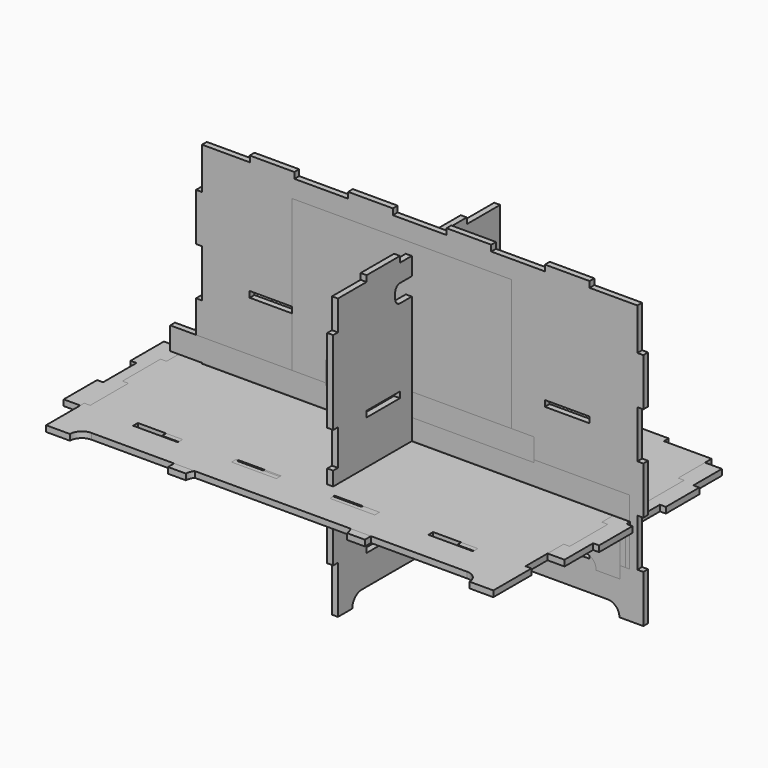
from build123d import *

# Parameters (mm, degrees)
F1_DEPTH  = 12.7
F3_DEPTH  = 12.7
F4_W      = 95.25
F4_H      = 12.7
F4_H_2    = 12.3182607685
F5_DEPTH  = 12.7
F6_W      = 88.9
F6_H      = 12.7
F7_DEPTH  = 12.7
F9_DEPTH  = 12.7
F11_DEPTH = 12.7
F13_DEPTH = 12.7
F14_W     = 88.9
F14_H     = 12.7
F15_DEPTH = 12.7
F16_W     = 95.25
F16_H     = 12.7
F16_H_2   = 12.3182607685
F17_DEPTH = 12.7
F18_W     = 467.36
F18_H     = 482.6
F19_DEPTH = 12.7
F18_W_2   = 15.24
F20_DEPTH = 6.35
F21_W     = 977.9
F21_H     = 48.26
F22_DEPTH = 12.7
F23_W     = 444.5
F23_H     = 48.26
F24_DEPTH = 12.7


with BuildPart() as f1:
    # F0 (on Top) → F1 (new body)
    with BuildSketch(Plane.XY):
        Polygon((-533.4, -256.6132211758), (-520.7, -256.6132211758), (-419.1, -256.6132211758), (-419.1, -243.9132211758), (-323.85, -243.9132211758), (-323.85, -256.6132211758), (-209.55, -256.6132211758), (-209.55, -243.9132211758), (-114.3, -243.9132211758), (-114.3, -256.6132211758), (0, -256.6132211758), (0, -243.9132211758), (95.25, -243.9132211758), (95.25, -256.6132211758), (209.55, -256.6132211758), (209.55, -243.9132211758), (304.8, -243.9132211758), (304.8, -256.6132211758), (406.4, -256.6132211758), (419.1, -256.6132211758), (419.1, -167.7132211758), (406.4, -167.7132211758), (406.4, -79.9850564738), (419.1, -79.9850564738), (419.1, 10.0867788242), (406.4, 10.0867788242), (406.4, 98.9867788242), (419.1, 98.9867788242), (419.1, 187.8867788242), (304.8, 187.8867788242), (304.8, 175.1867788242), (209.55, 175.1867788242), (209.55, 187.8867788242), (95.25, 187.8867788242), (95.25, 175.1867788242), (0, 175.1867788242), (0, 187.8867788242), (-114.3, 187.8867788242), (-114.3, 175.1867788242), (-209.55, 175.1867788242), (-209.55, 187.8867788242), (-323.85, 187.8867788242), (-323.85, 175.1867788242), (-419.1, 175.1867788242), (-419.1, 187.8867788242), (-520.7, 187.8867788242), (-520.7, 187.8943966269), (-533.4, 187.8943966269), (-533.4, 98.9943966269), (-520.7, 98.9943966269), (-520.7, 10.0943966269), (-533.4, 10.0943966269), (-533.4, -78.8056033731), (-520.7, -78.8056033731), (-520.7, -167.7132211758), (-533.4, -167.7132211758), align=None)
    extrude(amount=F1_DEPTH)


with BuildPart() as f3:
    # F2 (on Top) → F3 (new body)
    with BuildSketch(Plane.XY):
        Polygon((-252.5200699091, 244.3481689453), (-347.7700699091, 244.3481689453), (-347.7700699091, 231.6481689453), (-449.3700699091, 231.6481689453), (-449.3700699091, 155.4481689453), (-462.0700699091, 155.4481689453), (-462.0700699091, 66.5481689453), (-449.3700699091, 66.5481689453), (-449.3700699091, -22.3518310547), (-462.0700699091, -22.3518310547), (-462.0700699091, -111.2518310547), (-449.3700699091, -111.2518310547), (-449.3700699091, -187.4518310547), (-347.7700699091, -187.4518310547), (-347.7700699091, -200.1518310547), (-252.5200699091, -200.1518310547), (-252.5200699091, -187.4518310547), (-138.2200699091, -187.4518310547), (-138.2200699091, -200.1518310547), (-42.9700699091, -200.1518310547), (-42.9700699091, -187.4518310547), (71.3299300909, -187.4518310547), (71.3299300909, -200.1518310547), (166.5799300909, -200.1518310547), (166.5799300909, -187.4518310547), (280.8799300909, -187.4518310547), (280.8799300909, -200.1518310547), (376.1299300909, -200.1518310547), (376.1299300909, -187.4518310547), (477.7299300909, -187.4518310547), (477.7299300909, -111.2518310547), (490.4299300909, -111.2518310547), (490.4299300909, -22.3518310547), (477.7299300909, -22.3518310547), (477.7299300909, 66.5481689453), (490.4299300909, 66.5481689453), (490.4299300909, 155.4481689453), (477.7299300909, 155.4481689453), (477.7299300909, 231.6481689453), (376.1299300909, 231.6481689453), (376.1299300909, 244.3481689453), (280.8799300909, 244.3481689453), (280.8799300909, 231.6481689453), (166.5799300909, 231.6481689453), (166.5799300909, 244.3481689453), (71.3299300909, 244.3481689453), (71.3299300909, 231.6481689453), (-42.9700699091, 231.6481689453), (-42.9700699091, 244.3481689453), (-138.2200699091, 244.3481689453), (-138.2200699091, 231.6481689453), (-252.5200699091, 231.6481689453), align=None)
    extrude(amount=F3_DEPTH)


with BuildPart() as f5:
    # F4 (on Front) → F5 (new body)
    with BuildSketch(Plane.XZ):
        with BuildLine():
            Line((-446.7179388881, -71.9391102995), (-446.7179388881, -173.5391102995))
            Line((-446.7179388881, -173.5391102995), (-395.9179388881, -173.5391102995))
            ThreePointArc((-395.9179388881, -173.5391102995), (-388.4784511302, -155.5785980574), (-370.5179388881, -148.1391102995))
            Line((-370.5179388881, -148.1391102995), (429.5820611119, -148.1391102995))
            ThreePointArc((429.5820611119, -148.1391102995), (447.5836700028, -155.619788958), (454.9817945276, -173.6554821625))
            Line((454.9817945276, -173.6554821625), (505.7820611119, -173.6554821625))
            Line((505.7820611119, -173.6554821625), (505.7820611119, -72.0554821625))
            Line((505.7820611119, -72.0554821625), (493.0820611119, -72.0554821625))
            Line((493.0820611119, -72.0554821625), (493.0820611119, 29.5445178375))
            Line((493.0820611119, 29.5445178375), (505.7820611119, 29.5445178375))
            Line((505.7820611119, 29.5445178375), (505.7820611119, 131.1445178375))
            Line((505.7820611119, 131.1445178375), (493.0820611119, 131.1445178375))
            Line((493.0820611119, 131.1445178375), (493.0820611119, 232.7445178375))
            Line((493.0820611119, 232.7445178375), (505.7820611119, 232.7445178375))
            Line((505.7820611119, 232.7445178375), (505.7820611119, 334.3445178375))
            Line((505.7820611119, 334.3445178375), (493.0820611119, 334.3445178375))
            Line((493.0820611119, 334.3445178375), (493.0820611119, 423.3608897005))
            Line((493.0820611119, 423.3608897005), (391.4820611119, 423.3608897005))
            Line((391.4820611119, 423.3608897005), (391.4820611119, 436.0608897005))
            Line((391.4820611119, 436.0608897005), (296.2320611119, 436.0608897005))
            Line((296.2320611119, 436.0608897005), (296.2320611119, 423.2445178375))
            Line((296.2320611119, 423.2445178375), (181.9320611119, 423.2445178375))
            Line((181.9320611119, 423.2445178375), (181.9320611119, 436.0608897005))
            Line((181.9320611119, 436.0608897005), (86.6820611119, 436.0608897005))
            Line((86.6820611119, 436.0608897005), (86.6820611119, 423.2445178375))
            Line((86.6820611119, 423.2445178375), (-27.6179388881, 423.2445178375))
            Line((-27.6179388881, 423.2445178375), (-27.6179388881, 436.0608897005))
            Line((-27.6179388881, 436.0608897005), (-122.8679388881, 436.0608897005))
            Line((-122.8679388881, 436.0608897005), (-122.8679388881, 423.2445178375))
            Line((-122.8679388881, 423.2445178375), (-237.1679388881, 423.2445178375))
            Line((-237.1679388881, 423.2445178375), (-237.1679388881, 436.0608897005))
            Line((-237.1679388881, 436.0608897005), (-332.4179388881, 436.0608897005))
            Line((-332.4179388881, 436.0608897005), (-331.8523272631, 423.3608897005))
            Line((-331.8523272631, 423.3608897005), (-434.0179388881, 423.3608897005))
            Line((-434.0179388881, 423.3608897005), (-434.0179388881, 334.4608897005))
            Line((-434.0179388881, 334.4608897005), (-446.7179388881, 334.4608897005))
            Line((-446.7179388881, 334.4608897005), (-446.7179388881, 232.8608897005))
            Line((-446.7179388881, 232.8608897005), (-434.0179388881, 232.8608897005))
            Line((-434.0179388881, 232.8608897005), (-434.0179388881, 131.2608897005))
            Line((-434.0179388881, 131.2608897005), (-446.7179388881, 131.2608897005))
            Line((-446.7179388881, 131.2608897005), (-446.7179388881, 29.6608897005))
            Line((-446.7179388881, 29.6608897005), (-434.0179388881, 29.6608897005))
            Line((-434.0179388881, 29.6608897005), (-434.0179388881, -71.9391102995))
            Line((-434.0179388881, -71.9391102995), (-446.7179388881, -71.9391102995))
        make_face()
        with Locations((-284.7929388881, -78.2891102995)):
            Rectangle(F4_W, F4_H, mode=Mode.SUBTRACT)
        with Locations((-75.2429388881, -78.2891102995)):
            Rectangle(F4_W, F4_H, mode=Mode.SUBTRACT)
        with Locations((134.3070611119, -78.2891102995)):
            Rectangle(F4_W, F4_H, mode=Mode.SUBTRACT)
        with Locations((343.8570611119, -78.2891102995)):
            Rectangle(F4_W, F4_H, mode=Mode.SUBTRACT)
        with Locations((-284.7929388881, 175.7108897005)):
            Rectangle(F4_W, F4_H, mode=Mode.SUBTRACT)
        with Locations((-75.2429388881, 175.9017593162)):
            Rectangle(F4_W, F4_H_2, mode=Mode.SUBTRACT)
        with Locations((134.3070611119, 175.7108897005)):
            Rectangle(F4_W, F4_H, mode=Mode.SUBTRACT)
        with Locations((343.8570611119, 175.7108897005)):
            Rectangle(F4_W, F4_H, mode=Mode.SUBTRACT)
    extrude(amount=F5_DEPTH)


with BuildPart() as f7:
    # F6 (on Right) → F7 (new body)
    with BuildSketch(Plane.YZ):
        with BuildLine():
            Line((-44.0499485254, 372.7201488963), (-132.9499485254, 372.7201488963))
            Line((-132.9499485254, 372.7201488963), (-132.9499485254, 360.0201488963))
            Line((-132.9499485254, 360.0201488963), (-209.1499485254, 360.0201488963))
            Line((-209.1499485254, 360.0201488963), (-209.1499485254, 296.5201488963))
            Line((-209.1499485254, 296.5201488963), (-221.8499485254, 296.5201488963))
            Line((-221.8499485254, 296.5201488963), (-221.8499485254, 118.7201488963))
            Line((-221.8499485254, 118.7201488963), (-209.1499485254, 118.7201488963))
            Line((-209.1499485254, 118.7201488963), (-209.1499485254, 42.5201488963))
            Line((-209.1499485254, 42.5201488963), (-221.8499485254, 42.5201488963))
            Line((-221.8499485254, 42.5201488963), (-221.8499485254, -135.2798511037))
            Line((-221.8499485254, -135.2798511037), (-209.1499485254, -135.2798511037))
            Line((-209.1499485254, -135.2798511037), (-209.1499485254, -236.8798511037))
            Line((-209.1499485254, -236.8798511037), (-171.0499485254, -236.8798511037))
            ThreePointArc((-171.0499485254, -236.8798511037), (-163.6104607676, -218.9193388616), (-145.6499485254, -211.4798511037))
            Line((-145.6499485254, -211.4798511037), (146.4500514746, -211.4798511037))
            ThreePointArc((146.4500514746, -211.4798511037), (164.4105637167, -218.9193388616), (171.8500514746, -236.8798511037))
            Line((171.8500514746, -236.8798511037), (209.9500514746, -236.8798511037))
            Line((209.9500514746, -236.8798511037), (209.9500514746, -135.2798511037))
            Line((209.9500514746, -135.2798511037), (222.6500514746, -135.2798511037))
            Line((222.6500514746, -135.2798511037), (222.6500514746, -33.6798511037))
            Line((222.6500514746, -33.6798511037), (209.9500514746, -33.6798511037))
            Line((209.9500514746, -33.6798511037), (209.9500514746, 67.9201488963))
            Line((209.9500514746, 67.9201488963), (222.6500514746, 67.9201488963))
            Line((222.6500514746, 67.9201488963), (222.6500514746, 169.5201488963))
            Line((222.6500514746, 169.5201488963), (209.9500514746, 169.5201488963))
            Line((209.9500514746, 169.5201488963), (209.9500514746, 271.1201488963))
            Line((209.9500514746, 271.1201488963), (222.6500514746, 271.1201488963))
            Line((222.6500514746, 271.1201488963), (222.6500514746, 360.0201488963))
            Line((222.6500514746, 360.0201488963), (209.9500514746, 360.0201488963))
            Line((209.9500514746, 360.0201488963), (133.7500514746, 360.0201488963))
            Line((133.7500514746, 360.0201488963), (133.7500514746, 372.7201488963))
            Line((133.7500514746, 372.7201488963), (44.8500514746, 372.7201488963))
            Line((44.8500514746, 372.7201488963), (44.8500514746, 360.0201488963))
            Line((44.8500514746, 360.0201488963), (-44.0499485254, 360.0201488963))
            Line((-44.0499485254, 360.0201488963), (-44.0499485254, 372.7201488963))
        make_face()
        with Locations((-88.4999485254, -141.6298511037)):
            Rectangle(F6_W, F6_H, mode=Mode.SUBTRACT)
        with Locations((89.3000514746, -141.6298511037)):
            Rectangle(F6_W, F6_H, mode=Mode.SUBTRACT)
        with Locations((-88.4999485254, 112.3701488963)):
            Rectangle(F6_W, F6_H, mode=Mode.SUBTRACT)
        with BuildLine():
            ThreePointArc((-56.7499485254, 309.2201488963), (-53.0302046465, 318.2004050173), (-44.0499485254, 321.9201488963))
            Line((-44.0499485254, 321.9201488963), (44.8500514746, 321.9201488963))
            ThreePointArc((44.8500514746, 321.9201488963), (53.8303075956, 318.2004050173), (57.5500514746, 309.2201488963))
            Line((57.5500514746, 309.2201488963), (57.5500514746, 296.5201488963))
            ThreePointArc((57.5500514746, 296.5201488963), (53.8303075956, 287.5398927752), (44.8500514746, 283.8201488963))
            Line((44.8500514746, 283.8201488963), (-44.0499485254, 283.8201488963))
            ThreePointArc((-44.0499485254, 283.8201488963), (-53.0302046465, 287.5398927752), (-56.7499485254, 296.5201488963))
            Line((-56.7499485254, 296.5201488963), (-56.7499485254, 309.2201488963))
        make_face(mode=Mode.SUBTRACT)
        with Locations((89.3000514746, 112.3701488963)):
            Rectangle(F6_W, F6_H, mode=Mode.SUBTRACT)
    extrude(amount=F7_DEPTH)


with BuildPart() as f9:
    # F8 (on Front) → F9 (new body)
    with BuildSketch(Plane.XZ):
        Polygon((-266.7, 0), (-361.95, 0), (-361.95, -12.7), (-476.25, -12.7), (-476.25, -76.2), (476.25, -76.2), (476.25, -12.7), (361.95, -12.7), (361.95, 0), (266.7, 0), (266.7, -12.7), (152.4, -12.7), (152.4, 0), (57.15, 0), (57.15, -12.7), (-57.15, -12.7), (-57.15, 0), (-152.4, 0), (-152.4, -12.7), (-266.7, -12.7), align=None)
    extrude(amount=F9_DEPTH)


with BuildPart() as f11:
    # F10 (on Front) → F11 (new body)
    with BuildSketch(Plane.XZ):
        Polygon((-370.8327061987, 0), (-485.1327061987, 0), (-485.1327061987, -76.2), (467.3672938013, -76.2), (467.3672938013, 0), (353.0672938013, 0), (353.0672938013, -12.7), (257.8172938013, -12.7), (257.8172938013, 0), (143.5172938013, 0), (143.5172938013, -12.7), (48.2672938013, -12.7), (48.2672938013, 0), (-66.0327061987, 0), (-66.0327061987, -12.7), (-161.2827061987, -12.7), (-161.2827061987, 0), (-275.5827061987, 0), (-275.5827061987, -12.7), (-370.8327061987, -12.7), align=None)
    extrude(amount=F11_DEPTH)


with BuildPart() as f13:
    # F12 (on Front) → F13 (new body)
    with BuildSketch(Plane.XZ):
        with BuildLine():
            Line((-381.8506570854, 0), (-496.1506570854, 0))
            Line((-496.1506570854, 0), (-496.1506570854, -101.6))
            Line((-496.1506570854, -101.6), (-445.3506570854, -101.6))
            ThreePointArc((-445.3506570854, -101.6), (-437.9111693276, -83.6394877579), (-419.9506570854, -76.2))
            Line((-419.9506570854, -76.2), (380.1493429146, -76.2))
            ThreePointArc((380.1493429146, -76.2), (398.1098551567, -83.6394877579), (405.5493429146, -101.6))
            Line((405.5493429146, -101.6), (456.3493429146, -101.6))
            Line((456.3493429146, -101.6), (456.3493429146, 0))
            Line((456.3493429146, 0), (342.0493429146, 0))
            Line((342.0493429146, 0), (342.0493429146, -12.7))
            Line((342.0493429146, -12.7), (246.7993429146, -12.7))
            Line((246.7993429146, -12.7), (246.7993429146, 0))
            Line((246.7993429146, 0), (132.4993429146, 0))
            Line((132.4993429146, 0), (132.4993429146, -12.7))
            Line((132.4993429146, -12.7), (37.2493429146, -12.7))
            Line((37.2493429146, -12.7), (37.2493429146, 0))
            Line((37.2493429146, 0), (-77.0506570854, 0))
            Line((-77.0506570854, 0), (-77.0506570854, -12.7))
            Line((-77.0506570854, -12.7), (-172.3006570854, -12.7))
            Line((-172.3006570854, -12.7), (-172.3006570854, 0))
            Line((-172.3006570854, 0), (-286.6006570854, 0))
            Line((-286.6006570854, 0), (-286.6006570854, -12.7))
            Line((-286.6006570854, -12.7), (-381.8506570854, -12.7))
            Line((-381.8506570854, -12.7), (-381.8506570854, 0))
        make_face()
    extrude(amount=F13_DEPTH)


with BuildPart() as f15:
    # F14 (on Top) → F15 (new body)
    with BuildSketch(Plane.XY):
        with BuildLine():
            Line((-80.5845238095, 271.1530918519), (-169.4845238095, 271.1530918519))
            Line((-169.4845238095, 271.1530918519), (-169.4845238095, 258.4530918519))
            Line((-169.4845238095, 258.4530918519), (-245.6845238095, 258.4530918519))
            Line((-245.6845238095, 258.4530918519), (-245.6845238095, 194.9530918519))
            Line((-245.6845238095, 194.9530918519), (-258.3845238095, 194.9530918519))
            Line((-258.3845238095, 194.9530918519), (-258.3845238095, 17.1530918519))
            Line((-258.3845238095, 17.1530918519), (-245.6845238095, 17.1530918519))
            Line((-245.6845238095, 17.1530918519), (-245.6845238095, -59.0469081481))
            Line((-245.6845238095, -59.0469081481), (-258.3845238095, -59.0469081481))
            Line((-258.3845238095, -59.0469081481), (-258.3845238095, -236.8469081481))
            Line((-258.3845238095, -236.8469081481), (-245.6845238095, -236.8469081481))
            Line((-245.6845238095, -236.8469081481), (-245.6845238095, -338.4469081481))
            Line((-245.6845238095, -338.4469081481), (-207.5845238095, -338.4469081481))
            ThreePointArc((-207.5845238095, -338.4469081481), (-200.1450360517, -320.4863959059), (-182.1845238095, -313.0469081481))
            Line((-182.1845238095, -313.0469081481), (109.9154761905, -313.0469081481))
            ThreePointArc((109.9154761905, -313.0469081481), (127.8759884326, -320.4863959059), (135.3154761905, -338.4469081481))
            Line((135.3154761905, -338.4469081481), (173.4154761905, -338.4469081481))
            Line((173.4154761905, -338.4469081481), (173.4154761905, -236.8469081481))
            Line((173.4154761905, -236.8469081481), (186.1154761905, -236.8469081481))
            Line((186.1154761905, -236.8469081481), (186.1154761905, -135.2469081481))
            Line((186.1154761905, -135.2469081481), (173.4154761905, -135.2469081481))
            Line((173.4154761905, -135.2469081481), (173.4154761905, -33.6469081481))
            Line((173.4154761905, -33.6469081481), (186.1154761905, -33.6469081481))
            Line((186.1154761905, -33.6469081481), (186.1154761905, 67.9530918519))
            Line((186.1154761905, 67.9530918519), (173.4154761905, 67.9530918519))
            Line((173.4154761905, 67.9530918519), (173.4154761905, 169.5530918519))
            Line((173.4154761905, 169.5530918519), (186.1154761905, 169.5530918519))
            Line((186.1154761905, 169.5530918519), (186.1154761905, 258.4530918519))
            Line((186.1154761905, 258.4530918519), (173.4154761905, 258.4530918519))
            Line((173.4154761905, 258.4530918519), (97.2154761905, 258.4530918519))
            Line((97.2154761905, 258.4530918519), (97.2154761905, 271.1530918519))
            Line((97.2154761905, 271.1530918519), (8.3154761905, 271.1530918519))
            Line((8.3154761905, 271.1530918519), (8.3154761905, 258.4530918519))
            Line((8.3154761905, 258.4530918519), (-80.5845238095, 258.4530918519))
            Line((-80.5845238095, 258.4530918519), (-80.5845238095, 271.1530918519))
        make_face()
        with Locations((-125.0345238095, -243.1969081481)):
            Rectangle(F14_W, F14_H, mode=Mode.SUBTRACT)
        with Locations((52.7654761905, -243.1969081481)):
            Rectangle(F14_W, F14_H, mode=Mode.SUBTRACT)
        with Locations((-125.0345238095, 10.8030918519)):
            Rectangle(F14_W, F14_H, mode=Mode.SUBTRACT)
        with BuildLine():
            ThreePointArc((-93.2845238095, 207.6530918519), (-89.5647799306, 216.633347973), (-80.5845238095, 220.3530918519))
            Line((-80.5845238095, 220.3530918519), (8.3154761905, 220.3530918519))
            ThreePointArc((8.3154761905, 220.3530918519), (17.2957323115, 216.633347973), (21.0154761905, 207.6530918519))
            Line((21.0154761905, 207.6530918519), (21.0154761905, 194.9530918519))
            ThreePointArc((21.0154761905, 194.9530918519), (17.2957323115, 185.9728357309), (8.3154761905, 182.2530918519))
            Line((8.3154761905, 182.2530918519), (-80.5845238095, 182.2530918519))
            ThreePointArc((-80.5845238095, 182.2530918519), (-89.5647799306, 185.9728357309), (-93.2845238095, 194.9530918519))
            Line((-93.2845238095, 194.9530918519), (-93.2845238095, 207.6530918519))
        make_face(mode=Mode.SUBTRACT)
        with Locations((52.7654761905, 10.8030918519)):
            Rectangle(F14_W, F14_H, mode=Mode.SUBTRACT)
    extrude(amount=F15_DEPTH)


with BuildPart() as f17:
    # F16 (on Top) → F17 (new body)
    with BuildSketch(Plane.XY):
        with BuildLine():
            Line((-498.1293674064, -245.9926323121), (-498.1293674064, -347.5926323121))
            Line((-498.1293674064, -347.5926323121), (-447.3293674064, -347.5926323121))
            ThreePointArc((-447.3293674064, -347.5926323121), (-439.8898796485, -329.6321200699), (-421.9293674064, -322.1926323121))
            Line((-421.9293674064, -322.1926323121), (378.1706325936, -322.1926323121))
            ThreePointArc((378.1706325936, -322.1926323121), (396.1722414845, -329.6733109706), (403.5703660093, -347.7090041751))
            Line((403.5703660093, -347.7090041751), (454.3706325936, -347.7090041751))
            Line((454.3706325936, -347.7090041751), (454.3706325936, -246.1090041751))
            Line((454.3706325936, -246.1090041751), (441.6706325936, -246.1090041751))
            Line((441.6706325936, -246.1090041751), (441.6706325936, -144.5090041751))
            Line((441.6706325936, -144.5090041751), (454.3706325936, -144.5090041751))
            Line((454.3706325936, -144.5090041751), (454.3706325936, -42.9090041751))
            Line((454.3706325936, -42.9090041751), (441.6706325936, -42.9090041751))
            Line((441.6706325936, -42.9090041751), (441.6706325936, 58.6909958249))
            Line((441.6706325936, 58.6909958249), (454.3706325936, 58.6909958249))
            Line((454.3706325936, 58.6909958249), (454.3706325936, 160.2909958249))
            Line((454.3706325936, 160.2909958249), (441.6706325936, 160.2909958249))
            Line((441.6706325936, 160.2909958249), (441.6706325936, 249.3073676879))
            Line((441.6706325936, 249.3073676879), (340.0706325936, 249.3073676879))
            Line((340.0706325936, 249.3073676879), (340.0706325936, 262.0073676879))
            Line((340.0706325936, 262.0073676879), (244.8206325936, 262.0073676879))
            Line((244.8206325936, 262.0073676879), (244.8206325936, 249.1909958249))
            Line((244.8206325936, 249.1909958249), (130.5206325936, 249.1909958249))
            Line((130.5206325936, 249.1909958249), (130.5206325936, 262.0073676879))
            Line((130.5206325936, 262.0073676879), (35.2706325936, 262.0073676879))
            Line((35.2706325936, 262.0073676879), (35.2706325936, 249.1909958249))
            Line((35.2706325936, 249.1909958249), (-79.0293674064, 249.1909958249))
            Line((-79.0293674064, 249.1909958249), (-79.0293674064, 262.0073676879))
            Line((-79.0293674064, 262.0073676879), (-174.2793674064, 262.0073676879))
            Line((-174.2793674064, 262.0073676879), (-174.2793674064, 249.1909958249))
            Line((-174.2793674064, 249.1909958249), (-288.5793674064, 249.1909958249))
            Line((-288.5793674064, 249.1909958249), (-288.5793674064, 262.0073676879))
            Line((-288.5793674064, 262.0073676879), (-383.8293674064, 262.0073676879))
            Line((-383.8293674064, 262.0073676879), (-383.2637557814, 249.3073676879))
            Line((-383.2637557814, 249.3073676879), (-485.4293674064, 249.3073676879))
            Line((-485.4293674064, 249.3073676879), (-485.4293674064, 160.4073676879))
            Line((-485.4293674064, 160.4073676879), (-498.1293674064, 160.4073676879))
            Line((-498.1293674064, 160.4073676879), (-498.1293674064, 58.8073676879))
            Line((-498.1293674064, 58.8073676879), (-485.4293674064, 58.8073676879))
            Line((-485.4293674064, 58.8073676879), (-485.4293674064, -42.7926323121))
            Line((-485.4293674064, -42.7926323121), (-498.1293674064, -42.7926323121))
            Line((-498.1293674064, -42.7926323121), (-498.1293674064, -144.3926323121))
            Line((-498.1293674064, -144.3926323121), (-485.4293674064, -144.3926323121))
            Line((-485.4293674064, -144.3926323121), (-485.4293674064, -245.9926323121))
            Line((-485.4293674064, -245.9926323121), (-498.1293674064, -245.9926323121))
        make_face()
        with Locations((-336.2043674064, -252.3426323121)):
            Rectangle(F16_W, F16_H, mode=Mode.SUBTRACT)
        with Locations((-126.6543674064, -252.3426323121)):
            Rectangle(F16_W, F16_H, mode=Mode.SUBTRACT)
        with Locations((82.8956325936, -252.3426323121)):
            Rectangle(F16_W, F16_H, mode=Mode.SUBTRACT)
        with Locations((292.4456325936, -252.3426323121)):
            Rectangle(F16_W, F16_H, mode=Mode.SUBTRACT)
        with Locations((-336.2043674064, 1.6573676879)):
            Rectangle(F16_W, F16_H, mode=Mode.SUBTRACT)
        with Locations((-126.6543674064, 1.8482373037)):
            Rectangle(F16_W, F16_H_2, mode=Mode.SUBTRACT)
        with Locations((82.8956325936, 1.6573676879)):
            Rectangle(F16_W, F16_H, mode=Mode.SUBTRACT)
        with Locations((292.4456325936, 1.6573676879)):
            Rectangle(F16_W, F16_H, mode=Mode.SUBTRACT)
    extrude(amount=F17_DEPTH)


with BuildPart() as f19:
    # F18 (on Front) → F19 (new body)
    with BuildSketch(Plane.XZ):
        with Locations((-8.5534459901, 143.4637940012)):
            Rectangle(F18_W, F18_H)
    extrude(amount=F19_DEPTH)

    # F18 (on Front) → F20 (join)
    with BuildSketch(Plane.XZ):
        with Locations((232.7465540099, 143.4637940012)):
            Rectangle(F18_W_2, F18_H)
    extrude(amount=F20_DEPTH)


with BuildPart() as f22:
    # F21 (on Front) → F22 (new body)
    with BuildSketch(Plane.XZ):
        with Locations((-12.7571374178, 38.42341147)):
            Rectangle(F21_W, F21_H)
    extrude(amount=F22_DEPTH)


with BuildPart() as f24:
    # F23 (on Front) → F24 (new body)
    with BuildSketch(Plane.XZ):
        with Locations((51.0222762823, 81.2785354265)):
            Rectangle(F23_W, F23_H)
    extrude(amount=F24_DEPTH)


solid = Compound([f1.part, f3.part, f5.part, f7.part, f9.part, f11.part, f13.part, f15.part, f17.part, f19.part, f22.part, f24.part])
